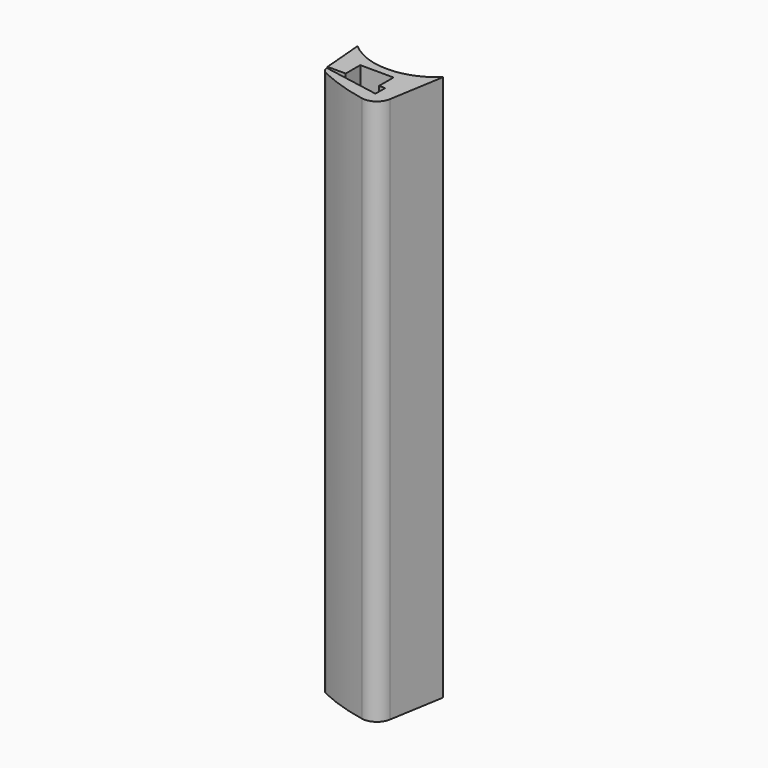
from build123d import *

# Parameters (mm, degrees)
F1_DEPTH    = 180
F2_R        = 5
F3_T1_DEPTH = 189.5214724234


# Not quite as in the source:
# - a fillet or chamfer that OpenCascade refuses, or shapes differently, is made with other operations: its cross-section is extruded or revolved along the edge and cut away or added


with BuildPart() as f1:
    # F0 (on Top) → F1 (new body)
    with BuildSketch(Plane.XY):
        with BuildLine():
            ThreePointArc((14.1226732436, -15.5418821401), (0.1645874713, -20.9993550131), (-13.8773267564, -15.7613388421))
            Line((-13.8773267564, -15.7613388421), (-12.7134246975, -29.6120676683))
            Line((-12.7134246975, -29.6120676683), (-6.7134246975, -29.6071426253))
            Line((-6.7134246975, -29.6071426253), (-6.7134246975, -23.6071426253))
            Line((-6.7134246975, -23.6071426253), (4.2865298223, -23.6563930556))
            Line((4.2865298223, -23.6563930556), (4.2865298223, -29.6071426253))
            Line((4.2865298223, -29.6071426253), (6.2865237583, -29.6120676683))
            Line((6.2865237583, -29.6120676683), (6.2766736722, -33.6120555403))
            Line((6.2766736722, -33.6120555403), (-12.4721404439, -30.2120676683))
            Line((-12.4721404439, -30.2120676683), (-12.4721404439, -31.7862083661))
            ThreePointArc((-12.4721404439, -31.7862083661), (-1.3967093827, -36.1708063262), (10.2766736722, -38.5418821401))
            Line((10.2766736722, -38.5418821401), (14.1226732436, -15.5418821401))
        make_face()
    extrude(amount=F1_DEPTH)

    # F2
    f2_edges = [f1.edges().sort_by_distance(p)[0] for p in [
        (10.276674, -38.541882, 90),
    ]]
    fillet(f2_edges, radius=F2_R)

    # F3: fillet of radius 3 on 1 edges, made by hand

    # F3_s2 → F3_t1 (cut)
    with BuildSketch(Plane.XY.offset(-4.7607362117)):
        with BuildLine():
            ThreePointArc((-10.7583691092, -32.6164645294), (-11.9315343306, -31.6396992801), (-12.4721404439, -30.2120676683))
            Line((-12.4721404439, -30.2120676683), (-12.4721404439, -31.7862083661))
            ThreePointArc((-12.4721404439, -31.7862083661), (-11.618180513, -32.2073755998), (-10.7583691092, -32.6164645294))
        make_face()
    extrude(amount=F3_T1_DEPTH, mode=Mode.SUBTRACT)


solid = f1.part
